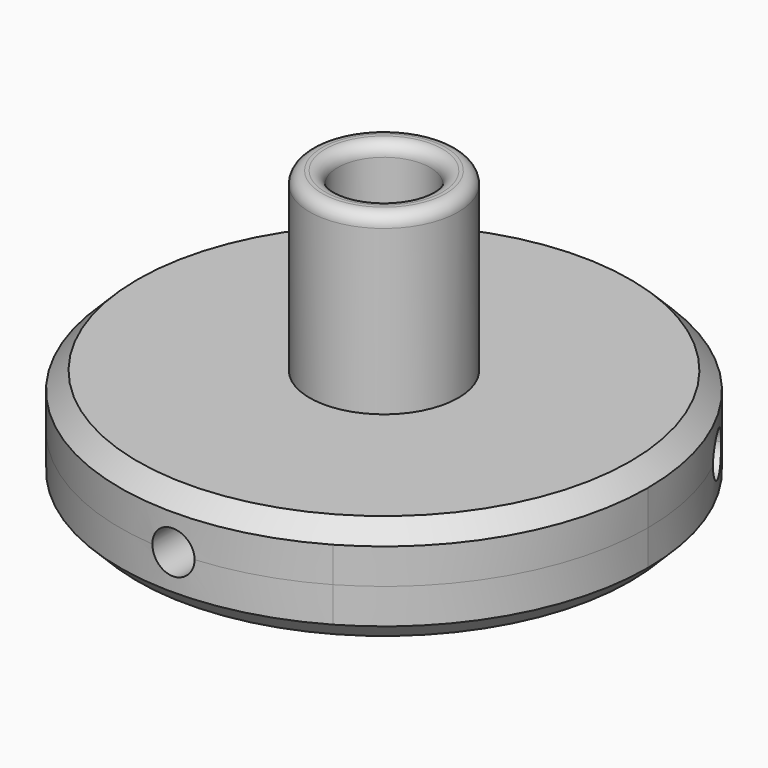
from build123d import *

# Parameters (mm, degrees)
F2_DEPTH = 25
F3_COUNT = 3
F4_DEPTH = 3
F6_R     = 4.225
F6_R_2   = 2.625
F7_DEPTH = 10
F9_DEPTH = 6
F10_R    = 0.7


# Not quite as in the source:
# - a fillet or chamfer that OpenCascade refuses, or shapes differently, is made with other operations: its cross-section is extruded or revolved along the edge and cut away or added


with BuildPart() as f2:
    # F1 (on Front) → F2 (new body)
    with BuildSketch(Plane.XZ):
        with BuildLine():
            ThreePointArc((0, 1.2), (-0.8485281374, -0.8485281374), (1.2, 0))
            ThreePointArc((1.2, 0), (0.8485281374, 0.8485281374), (0, 1.2))
        make_face()
    extrude(amount=F2_DEPTH)

    # F3: F2 ×3 about axis
    f3_axis = Axis((0, 0, 16.2680745125), (0, 0, 1))


with BuildPart() as f2_1:
    add(f2.part)
    for i in range(1, F3_COUNT):
        add(f2.part.rotate(f3_axis, i * 360 / F3_COUNT))


with BuildPart() as f4:
    # F0 (on Top) → F4 (new body, symmetric)
    with BuildSketch(Plane.XY):
        with BuildLine():
            Line((0, 0), (7.5, 12.9903810568))
            ThreePointArc((7.5, 12.9903810568), (-7.5, 12.9903810568), (-15, 0))
            Line((-15, 0), (0, 0))
        make_face()
        with BuildLine():
            ThreePointArc((-15, 0), (-7.5, -12.9903810568), (7.5, -12.9903810568))
            Line((7.5, -12.9903810568), (0, 0))
            Line((0, 0), (-15, 0))
        make_face()
        with BuildLine():
            ThreePointArc((7.5, -12.9903810568), (12.9903810568, -7.5), (15, 0))
            ThreePointArc((15, 0), (12.9903810568, 7.5), (7.5, 12.9903810568))
            Line((7.5, 12.9903810568), (0, 0))
            Line((0, 0), (7.5, -12.9903810568))
        make_face()
        with BuildLine():
            Line((0, 0), (7.5, 12.9903810568))
            ThreePointArc((7.5, 12.9903810568), (-7.5, 12.9903810568), (-15, 0))
            Line((-15, 0), (0, 0))
        make_face()
        with BuildLine():
            ThreePointArc((-15, 0), (-7.5, -12.9903810568), (7.5, -12.9903810568))
            Line((7.5, -12.9903810568), (0, 0))
            Line((0, 0), (-15, 0))
        make_face()
        with BuildLine():
            ThreePointArc((7.5, -12.9903810568), (12.9903810568, -7.5), (15, 0))
            ThreePointArc((15, 0), (12.9903810568, 7.5), (7.5, 12.9903810568))
            Line((7.5, 12.9903810568), (0, 0))
            Line((0, 0), (7.5, -12.9903810568))
        make_face()
    extrude(amount=F4_DEPTH, both=True)

    # F5: cut F2
    add(f2_1.part, mode=Mode.SUBTRACT)

    # F6 (on face) → F7 (join)
    with BuildSketch(Plane.XY.offset(3)):
        Circle(F6_R)
        Circle(F6_R_2, mode=Mode.SUBTRACT)
    extrude(amount=F7_DEPTH)

    # F8: chamfer of 1 on 2 edges, made by hand

    # F8_s1 → F8_t2 (revolve, cut)
    with BuildSketch(Plane.XZ):
        Polygon((-15, 2), (-14, 3), (-15, 3), align=None)
    revolve(axis=Axis((0, 0, 3), (0, 0, 1)), mode=Mode.SUBTRACT)

    # F8_s3 → F8_t4 (revolve, cut)
    with BuildSketch(Plane.XZ):
        Polygon((-15, -2), (-14, -3), (-15, -3), align=None)
    revolve(axis=Axis((0, 0, -3), (0, 0, 1)), mode=Mode.SUBTRACT)

    # F9 (add): a face of the model
    f9_faces = [f4.faces().sort_by_distance(p)[0] for p in [
        (0, 0, 3),
    ]]
    extrude(f9_faces, amount=-F9_DEPTH)

    # F10
    f10_edges = [f4.edges().sort_by_distance(p)[0] for p in [
        (-2.625, 0, 13),
        (-4.225, 0, 13),
    ]]
    fillet(f10_edges, radius=F10_R)


solid = f4.part
